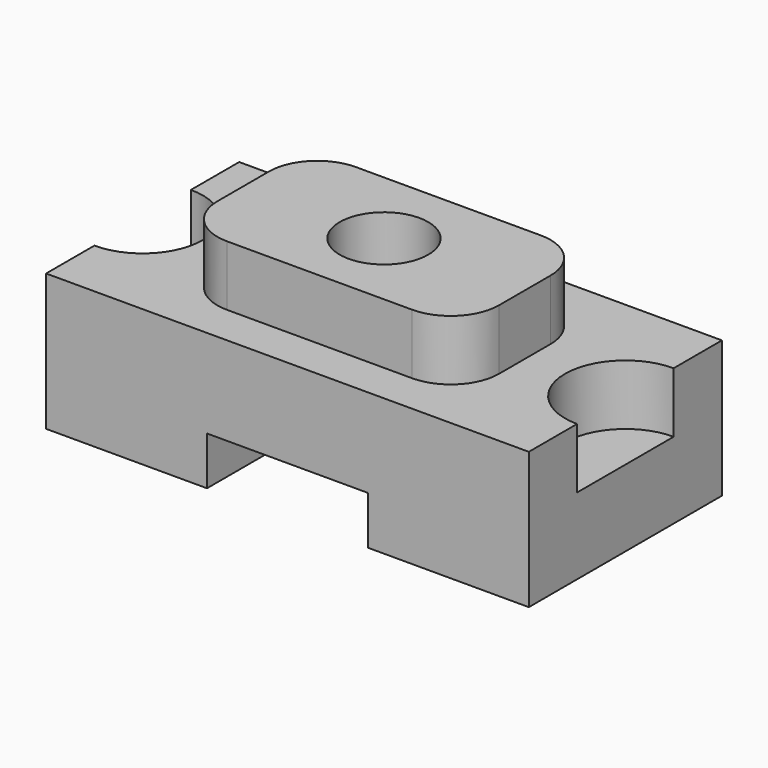
from build123d import *

# Parameters (mm, degrees)
F0_W     = 1200
F0_H     = 340
F1_DEPTH = 600
F3_DEPTH = 150
F4_W     = 400
F4_H     = 120
F5_DEPTH = 600.001
F7_DEPTH = 150
F8_R     = 110
F9_DEPTH = 490.001


# Not quite as in the source:
# - a feature names something its author has since deleted; it is built from what else it names


with BuildPart() as f1:
    # F0 (on Front) → F1 (new body)
    with BuildSketch(Plane.XZ):
        Rectangle(F0_W, F0_H)
    extrude(amount=F1_DEPTH)

    # F2 (on face) → F3 (cut)
    with BuildSketch(Plane.XY.offset(170)):
        with BuildLine():
            Line((-600, -150), (-600, -450))
            ThreePointArc((-600, -450), (-450, -300), (-600, -150))
        make_face()
        with BuildLine():
            ThreePointArc((600, -150), (450, -300), (600, -450))
            Line((600, -450), (600, -150))
        make_face()
    extrude(amount=-F3_DEPTH, mode=Mode.SUBTRACT)

    # F4 (on face) → F5 (cut, through all)
    with BuildSketch(Plane(origin=(0, 0, 0), x_dir=(-1, 0, 0), z_dir=(0, 1, 0))):
        with Locations((0, -110)):
            Rectangle(F4_W, F4_H)
    extrude(amount=-F5_DEPTH, mode=Mode.SUBTRACT)

    # F6 (on face) → F7 (join)
    with BuildSketch(Plane.XY.offset(170)):
        with BuildLine():
            Line((230, -100), (-230, -100))
            ThreePointArc((-230, -100), (-314.8528137424, -135.1471862576), (-350, -220))
            Line((-350, -220), (-350, -380))
            ThreePointArc((-350, -380), (-314.8528137424, -464.8528137424), (-230, -500))
            Line((-230, -500), (230, -500))
            ThreePointArc((230, -500), (314.8528137424, -464.8528137424), (350, -380))
            Line((350, -380), (350, -220))
            ThreePointArc((350, -220), (314.8528137424, -135.1471862576), (230, -100))
        make_face()
    extrude(amount=F7_DEPTH)

    # F8 (on face) → F9 (cut, through all)
    with BuildSketch(Plane.XY.offset(320)):
        with Locations((0, -300)):
            Circle(F8_R)
    extrude(amount=-F9_DEPTH, mode=Mode.SUBTRACT)


solid = f1.part
